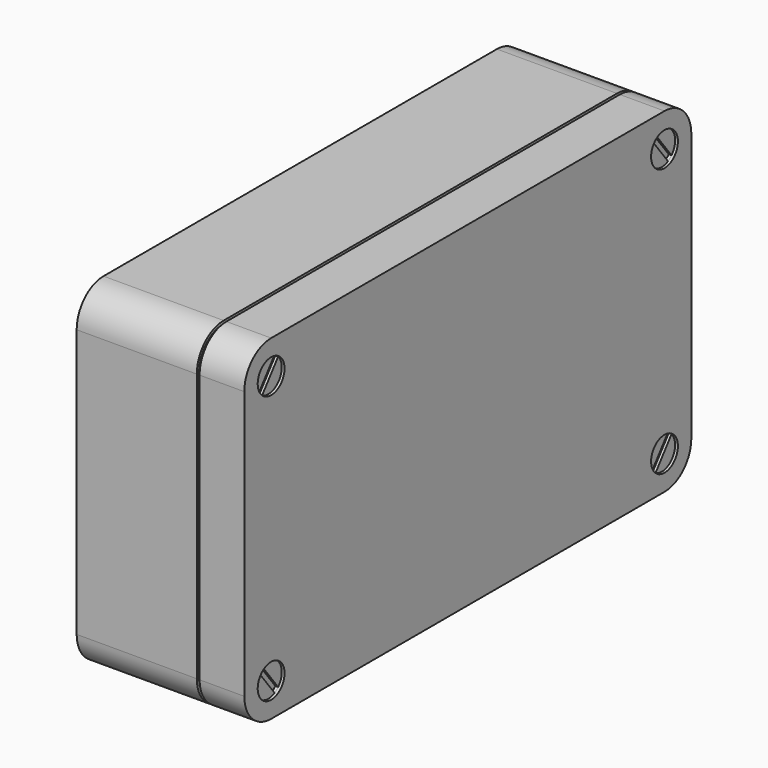
from build123d import *

# Parameters (mm, degrees)
F0_W             = 200
F0_H             = 120
F1_DEPTH         = 60
F2_R             = 12
F5_DEPTH         = 1
F6_R             = 6
F7_DEPTH         = 1
F7_COPIES2_COUNT = 2
F7_COPIES2_PITCH = 200.479425
F9_DEPTH         = 1
F9_COPIES2_COUNT = 2
F9_COPIES2_PITCH = 200.479425


# Not quite as in the source:
# - a pattern or mirror of a feature is missing from the dataset's text; its kind, count and spacing are read off the source's solid


with BuildPart() as f1:
    # F0 (on Right) → F1 (new body)
    with BuildSketch(Plane.YZ):
        Rectangle(F0_W, F0_H)
    extrude(amount=-F1_DEPTH)

    # F2
    f2_edges = [f1.edges().sort_by_distance(p)[0] for p in [
        (-30, -100, 60),
        (-30, -100, -60),
        (-30, 100, -60),
        (-30, 100, 60),
    ]]
    fillet(f2_edges, radius=F2_R)

    # F4 (on offset) → F5 (cut)
    with BuildSketch(Plane.YZ.offset(-16)):
        with BuildLine():
            ThreePointArc((-88, 60), (-96.4852813742, 56.4852813742), (-100, 48))
            Line((-100, 48), (-100, -48))
            ThreePointArc((-100, -48), (-96.4852813742, -56.4852813742), (-88, -60))
            Line((-88, -60), (88, -60))
            ThreePointArc((88, -60), (96.4852813742, -56.4852813742), (100, -48))
            Line((100, -48), (100, 48))
            ThreePointArc((100, 48), (96.4852813742, 56.4852813742), (88, 60))
            Line((88, 60), (-88, 60))
        make_face()
        with BuildLine():
            ThreePointArc((-99, 48), (-95.7781745931, 55.7781745931), (-88, 59))
            Line((-88, 59), (88, 59))
            ThreePointArc((88, 59), (95.7781745931, 55.7781745931), (99, 48))
            Line((99, 48), (99, -48))
            ThreePointArc((99, -48), (95.7781745931, -55.7781745931), (88, -59))
            Line((88, -59), (-88, -59))
            ThreePointArc((-88, -59), (-95.7781745931, -55.7781745931), (-99, -48))
            Line((-99, -48), (-99, 48))
        make_face(mode=Mode.SUBTRACT)
    extrude(amount=-F5_DEPTH, mode=Mode.SUBTRACT)

    # F6 (on face) → F7 (cut)
    with BuildSketch(Plane.YZ):
        with Locations((-88, 48)):
            Circle(F6_R)
    f7 = extrude(amount=-F7_DEPTH, mode=Mode.SUBTRACT)

    # F7_copies: F7 across plane
    add(f7.mirror(Plane.ZX), mode=Mode.SUBTRACT)

    # F7_copies1: F7 across plane
    add(f7.mirror(Plane(origin=(0, 0, 0), x_dir=(-1, 0, 0), z_dir=(0, 0, -1))), mode=Mode.SUBTRACT)

    # F7_copies2: F7 ×2
    with Locations(*[Vector(0, 0.8778955729, -0.4788521307) * (i * F7_COPIES2_PITCH) for i in range(1, F7_COPIES2_COUNT)]):
        add(f7, mode=Mode.SUBTRACT)

    # F8 (on face) → F9 (cut)
    with BuildSketch(Plane.YZ.offset(-1)):
        with BuildLine():
            Line((-90.8109403928, 42.6991874106), (-83.6029990627, 52.0824481328))
            ThreePointArc((-83.6029990627, 52.0824481328), (-84.3449066302, 52.7581816336), (-85.1890596072, 53.3008125894))
            Line((-85.1890596072, 53.3008125894), (-92.3970009373, 43.9175518672))
            ThreePointArc((-92.3970009373, 43.9175518672), (-91.6550933698, 43.2418183664), (-90.8109403928, 42.6991874106))
        make_face()
    f9 = extrude(amount=-F9_DEPTH, mode=Mode.SUBTRACT)

    # F9_copies: F9 across plane
    add(f9.mirror(Plane.ZX), mode=Mode.SUBTRACT)

    # F9_copies1: F9 across plane
    add(f9.mirror(Plane(origin=(0, 0, 0), x_dir=(-1, 0, 0), z_dir=(0, 0, -1))), mode=Mode.SUBTRACT)

    # F9_copies2: F9 ×2
    with Locations(*[Vector(0, 0.8778955729, -0.4788521307) * (i * F9_COPIES2_PITCH) for i in range(1, F9_COPIES2_COUNT)]):
        add(f9, mode=Mode.SUBTRACT)


solid = f1.part
